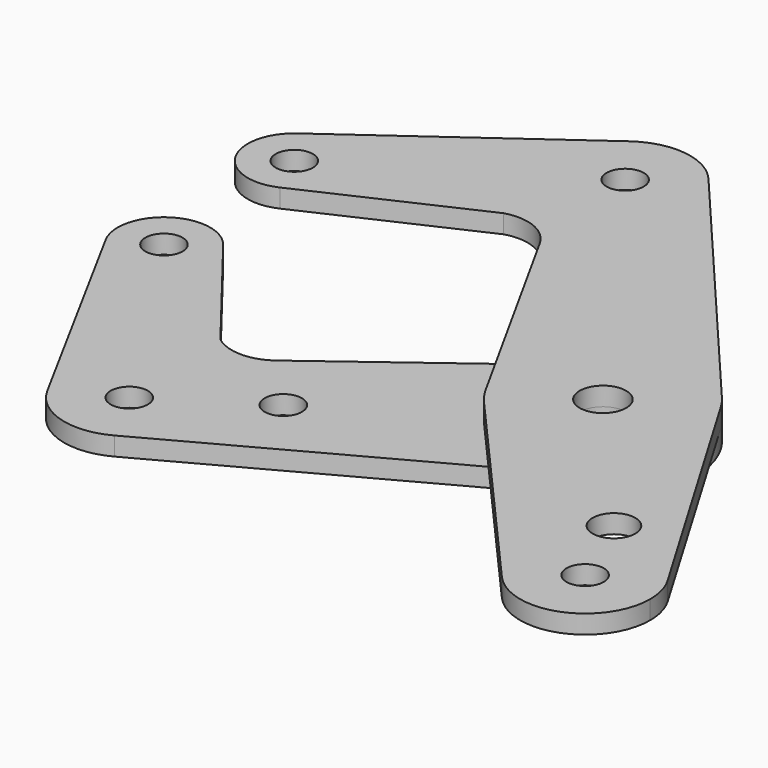
from build123d import *

# Parameters (mm, degrees)
F0_R     = 3.9751
F0_R_2   = 3.175
F1_DEPTH = 3.175
F2_DEPTH = 3.175


# Not quite as in the source:
# - a feature names something its author has since deleted; it is built from what else it names


with BuildPart() as f1:
    # F0 (on Top) → F1 (new body)
    with BuildSketch(Plane.XY):
        with BuildLine():
            ThreePointArc((-52.5748759492, 26.6492032122), (-53.8297565711, 22.3659212349), (-57.1976172398, 19.436971869))
            Line((-57.1976172398, 19.436971869), (-29.2551448321, 32.2793987644))
            ThreePointArc((-29.2551448321, 32.2793987644), (-23.9994310398, 32.0006966991), (-20.0694910529, 28.4998719382))
            Line((-20.0694910529, 28.4998719382), (-5.944542276, 2.9919030157))
            Line((-5.944542276, 2.9919030157), (5.1493091314, 11.2826215199))
            ThreePointArc((5.1493091314, 11.2826215199), (16.4418739956, 14.3401507274), (26.7626398944, 8.830858819))
            Line((26.7626398944, 8.830858819), (-14.1799710904, 57.1349621747))
            ThreePointArc((-14.1799710904, 57.1349621747), (-12.2239065675, 53.7759255754), (-11.5441699975, 49.9487499211))
            ThreePointArc((-11.5441699975, 49.9487499211), (-27.7288475633, 40.0587377986), (-29.1456623364, 58.9729854334))
            Line((-29.1456623364, 58.9729854334), (-65.0529744577, 33.1597232709))
            ThreePointArc((-65.0529744577, 33.1597232709), (-56.8406661575, 33.6864223686), (-52.5748759492, 26.6492032122))
        make_face()
        with BuildLine():
            Line((54.0656193027, -36.8819923981), (28.3160345311, 6.6486574689))
            ThreePointArc((28.3160345311, 6.6486574689), (29.9646775383, 2.7560340053), (30.5275292295, -1.4336842631))
            ThreePointArc((30.5275292295, -1.4336842631), (28.2876322337, -9.5638497635), (22.2000216938, -15.3997496539))
            Line((22.2000216938, -15.3997496539), (11.0862799953, -21.4057992729))
            Line((11.0862799953, -21.4057992729), (36.1609723562, -49.8832569445))
            ThreePointArc((36.1609723562, -49.8832569445), (33.6536306121, -40.1274456475), (40.059076729, -32.3535870991))
            ThreePointArc((40.059076729, -32.3535870991), (47.9196841374, -31.9660141026), (54.0656193027, -36.8819923981))
        make_face()
        with BuildLine():
            ThreePointArc((42.2477037346, -29.0114467929), (41.6518612023, -31.0089446024), (40.059076729, -32.3535870991))
            ThreePointArc((40.059076729, -32.3535870991), (35.5513078202, -27.0139489834), (42.2477037346, -29.0114467929))
        make_face(mode=Mode.SUBTRACT)
        with BuildLine():
            ThreePointArc((28.3160345311, 6.6486574689), (27.5854454003, 7.7725801433), (26.7626398944, 8.830858819))
            ThreePointArc((26.7626398944, 8.830858819), (16.4418739956, 14.3401507274), (5.1493091314, 11.2826215199))
            ThreePointArc((5.1493091314, 11.2826215199), (-0.8682400489, 1.9011839514), (0.7646299709, -9.1240600136))
            ThreePointArc((0.7646299709, -9.1240600136), (1.6755313717, -10.5777069884), (2.7379674647, -11.9245775975))
            ThreePointArc((2.7379674647, -11.9245775975), (11.8620044089, -17.0614990888), (22.2000216938, -15.3997496539))
            ThreePointArc((22.2000216938, -15.3997496539), (28.2876322337, -9.5638497635), (30.5275292295, -1.4336842631))
            ThreePointArc((30.5275292295, -1.4336842631), (29.9646775383, 2.7560340053), (28.3160345311, 6.6486574689))
        make_face()
        with Locations((14.6525292295, -1.4336842631)):
            Circle(F0_R, mode=Mode.SUBTRACT)
        with BuildLine():
            ThreePointArc((55.6136655916, -42.5396316105), (55.2196694077, -39.6068288226), (54.0656193027, -36.8819923981))
            ThreePointArc((54.0656193027, -36.8819923981), (47.9196841374, -31.9660141026), (40.059076729, -32.3535870991))
            ThreePointArc((40.059076729, -32.3535870991), (33.6536306121, -40.1274456475), (36.1609723562, -49.8832569445))
            ThreePointArc((36.1609723562, -49.8832569445), (48.4259113746, -52.9359784106), (55.6136655916, -42.5396316105))
        make_face()
        with Locations((44.5011655916, -42.5396316105)):
            Circle(F0_R_2, mode=Mode.SUBTRACT)
        with BuildLine():
            Line((5.1493091314, 11.2826215199), (-5.944542276, 2.9919030157))
            Line((-5.944542276, 2.9919030157), (0.7646299709, -9.1240600136))
            ThreePointArc((0.7646299709, -9.1240600136), (-0.8682400489, 1.9011839514), (5.1493091314, 11.2826215199))
        make_face()
        with BuildLine():
            ThreePointArc((22.2000216938, -15.3997496539), (11.8620044089, -17.0614990888), (2.7379674647, -11.9245775975))
            Line((2.7379674647, -11.9245775975), (11.0862799953, -21.4057992729))
            Line((11.0862799953, -21.4057992729), (22.2000216938, -15.3997496539))
        make_face()
        with BuildLine():
            ThreePointArc((-14.1799710904, 57.1349621747), (-21.3034591884, 60.9799616773), (-29.1456623364, 58.9729854334))
            ThreePointArc((-29.1456623364, 58.9729854334), (-27.7288475633, 40.0587377986), (-11.5441699975, 49.9487499211))
            ThreePointArc((-11.5441699975, 49.9487499211), (-12.2239065675, 53.7759255754), (-14.1799710904, 57.1349621747))
        make_face()
        with Locations((-22.6582662231, 49.9487499211)):
            Circle(F0_R_2, mode=Mode.SUBTRACT)
        with BuildLine():
            Line((-65.0529744577, 33.1597232709), (-65.2372085825, 33.0272799472))
            ThreePointArc((-65.2372085825, 33.0272799472), (-67.3440079309, 22.6078283574), (-57.1976172398, 19.436971869))
            ThreePointArc((-57.1976172398, 19.436971869), (-53.8297565711, 22.3659212349), (-52.5748759492, 26.6492032122))
            ThreePointArc((-52.5748759492, 26.6492032122), (-56.8406661575, 33.6864223686), (-65.0529744577, 33.1597232709))
        make_face()
        with Locations((-60.5123759492, 26.6492032122)):
            Circle(F0_R_2, mode=Mode.SUBTRACT)
    extrude(amount=F1_DEPTH)


with BuildPart() as f2:
    # F0 (on Top) → F2 (new body)
    with BuildSketch(Plane.XY):
        with BuildLine():
            Line((0.7646299709, -9.1240600136), (-5.944542276, 2.9919030157))
            Line((-5.944542276, 2.9919030157), (-30.1699189245, -15.1123396928))
            ThreePointArc((-30.1699189245, -15.1123396928), (-34.9928458304, -16.6939584439), (-39.7898032928, -15.0352417962))
            Line((-39.7898032928, -15.0352417962), (-56.5640629887, 6.5293747809))
            ThreePointArc((-56.5640629887, 6.5293747809), (-55.3280021129, 4.2441334268), (-54.9005552207, 1.6814271055))
            ThreePointArc((-54.9005552207, 1.6814271055), (-60.8502677302, -5.9708830942), (-69.7329844925, -2.090899427))
            Line((-69.7329844925, -2.090899427), (-48.5523916303, -41.0375117468))
            ThreePointArc((-48.5523916303, -41.0375117468), (-41.5291855152, -24.9587969806), (-27.6776447878, -35.7284447066))
            ThreePointArc((-27.6776447878, -35.7284447066), (-29.2455726849, -41.419560557), (-33.5069000628, -45.5046904802))
            Line((-33.5069000628, -45.5046904802), (11.0862799953, -21.4057992729))
            Line((11.0862799953, -21.4057992729), (2.7379674647, -11.9245775975))
            ThreePointArc((2.7379674647, -11.9245775975), (1.6755313717, -10.5777069884), (0.7646299709, -9.1240600136))
        make_face()
        with Locations((-21.4105871974, -24.5757886104)):
            Circle(F0_R_2, mode=Mode.SUBTRACT)
        with BuildLine():
            ThreePointArc((-54.9005552207, 1.6814271055), (-55.3280021129, 4.2441334268), (-56.5640629887, 6.5293747809))
            ThreePointArc((-56.5640629887, 6.5293747809), (-67.1209676687, 8.2878151961), (-69.7329844925, -2.090899427))
            ThreePointArc((-69.7329844925, -2.090899427), (-60.8502677302, -5.9708830942), (-54.9005552207, 1.6814271055))
        make_face()
        with Locations((-62.7964770983, 1.6814271055)):
            Circle(F0_R_2, mode=Mode.SUBTRACT)
        with BuildLine():
            ThreePointArc((-48.5523916303, -41.0375117468), (-41.9531001228, -46.3813020604), (-33.5069000628, -45.5046904802))
            ThreePointArc((-33.5069000628, -45.5046904802), (-29.2455726849, -41.419560557), (-27.6776447878, -35.7284447066))
            ThreePointArc((-27.6776447878, -35.7284447066), (-41.5291855152, -24.9587969806), (-48.5523916303, -41.0375117468))
        make_face()
        with Locations((-38.7901447878, -35.7284447066)):
            Circle(F0_R_2, mode=Mode.SUBTRACT)
        with BuildLine():
            Line((5.1493091314, 11.2826215199), (-5.944542276, 2.9919030157))
            Line((-5.944542276, 2.9919030157), (0.7646299709, -9.1240600136))
            ThreePointArc((0.7646299709, -9.1240600136), (-0.8682400489, 1.9011839514), (5.1493091314, 11.2826215199))
        make_face()
        with BuildLine():
            ThreePointArc((22.2000216938, -15.3997496539), (11.8620044089, -17.0614990888), (2.7379674647, -11.9245775975))
            Line((2.7379674647, -11.9245775975), (11.0862799953, -21.4057992729))
            Line((11.0862799953, -21.4057992729), (22.2000216938, -15.3997496539))
        make_face()
        with BuildLine():
            ThreePointArc((28.3160345311, 6.6486574689), (27.5854454003, 7.7725801433), (26.7626398944, 8.830858819))
            ThreePointArc((26.7626398944, 8.830858819), (16.4418739956, 14.3401507274), (5.1493091314, 11.2826215199))
            ThreePointArc((5.1493091314, 11.2826215199), (-0.8682400489, 1.9011839514), (0.7646299709, -9.1240600136))
            ThreePointArc((0.7646299709, -9.1240600136), (1.6755313717, -10.5777069884), (2.7379674647, -11.9245775975))
            ThreePointArc((2.7379674647, -11.9245775975), (11.8620044089, -17.0614990888), (22.2000216938, -15.3997496539))
            ThreePointArc((22.2000216938, -15.3997496539), (28.2876322337, -9.5638497635), (30.5275292295, -1.4336842631))
            ThreePointArc((30.5275292295, -1.4336842631), (29.9646775383, 2.7560340053), (28.3160345311, 6.6486574689))
        make_face()
        with Locations((14.6525292295, -1.4336842631)):
            Circle(F0_R, mode=Mode.SUBTRACT)
    extrude(amount=-F2_DEPTH)


solid = Compound([f1.part, f2.part])
